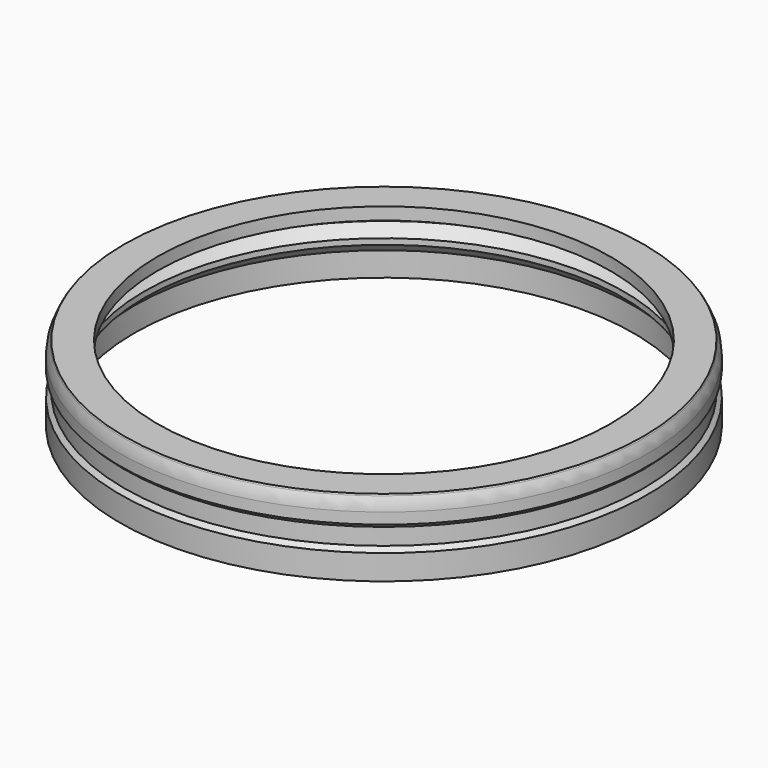
from build123d import *

# Parameters (mm, degrees)
F2_R = 3


# Not quite as in the source:
# - a feature names something its author has since deleted; it is built from what else it names


with BuildPart() as f1:
    # F0 (on Front) → F1 (revolve)
    with BuildSketch(Plane.XZ):
        Polygon((-30, 0.1), (-30, 3), (-28.8, 4.2), (-28.8, 4.9), (-30, 6.1), (-30, 7.6), (-27.2, 7.6), (-27.2, 9.1), (-31.2, 9.1), (-31.7, 8.2339745962), (-31.7, 6.1), (-31.2, 5.6), (-31.2, 3.6), (-31.7, 3.1), (-31.7, 0.1), align=None)
    revolve(axis=Axis((0, 0, 8.878365159), (0, 0, 1)))

    # F2
    f2_edges = [f1.edges().sort_by_distance(p)[0] for p in [
        (31.7, 0, 8.233975),
    ]]
    fillet(f2_edges, radius=F2_R)


solid = f1.part
